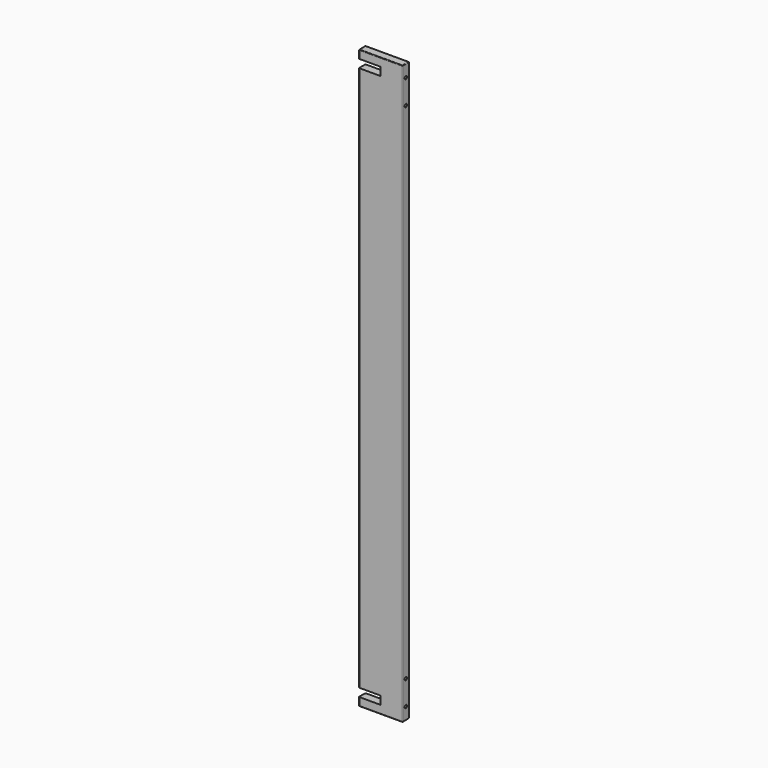
from build123d import *

# Parameters (mm, degrees)
F0_W     = 160
F0_H     = 30
F1_DEPTH = 1060
F2_R     = 2
F3_W     = 2
F3_H     = 30
F3_W_2   = 78
F4_DEPTH = 30.001
F3_W_3   = 80
F3_R     = 5.5
F5_DEPTH = 15
F6_R     = 5.5
F7_DEPTH = 15


# Not quite as in the source:
# - a pattern or mirror of a feature is missing from the dataset's text; its kind, count and spacing are read off the source's solid


with BuildPart() as f1:
    # F0 (on Top) → F1 (new body, symmetric)
    with BuildSketch(Plane.XY):
        Rectangle(F0_W, F0_H)
    extrude(amount=F1_DEPTH, both=True)

    # F2
    f2_edges = [f1.edges().sort_by_distance(p)[0] for p in [
        (0, -15, -1060),
        (80, -15, 0),
        (0, -15, 1060),
        (-80, -15, 0),
        (80, 15, 0),
        (0, 15, -1060),
        (-80, 15, 0),
        (0, 15, 1060),
        (80, 0, 1060),
        (-80, 0, 1060),
        (80, 0, -1060),
        (-80, 0, -1060),
    ]]
    fillet(f2_edges, radius=F2_R)

    # F3 (on face) → F4 (cut, through all)
    with BuildSketch(Plane(origin=(0, 15, 0), x_dir=(-1, 0, 0), z_dir=(0, 1, 0))):
        with Locations((79, 1015)):
            Rectangle(F3_W, F3_H)
        with Locations((39, 1015)):
            Rectangle(F3_W_2, F3_H)
        with Locations((79, -1015)):
            Rectangle(F3_W, F3_H)
        with Locations((39, -1015)):
            Rectangle(F3_W_2, F3_H)
    extrude(amount=-F4_DEPTH, mode=Mode.SUBTRACT)

    # F3 (on face) → F5 (cut)
    with BuildSketch(Plane(origin=(0, 15, 0), x_dir=(-1, 0, 0), z_dir=(0, 1, 0))):
        with Locations((40, 1015)):
            Rectangle(F3_W_3, F3_H)
        with Locations((40, -1015)):
            Rectangle(F3_W_3, F3_H)
        with Locations((25.4589803517, 924.7787594795)):
            Circle(F3_R)
    extrude(amount=-F5_DEPTH, mode=Mode.SUBTRACT)

    # F6 (on face) → F7 (cut)
    with BuildSketch(Plane.YZ.offset(80)):
        with Locations((0, 1015)):
            Circle(F6_R)
        with Locations((0, 925)):
            Circle(F6_R)
    f7 = extrude(amount=-F7_DEPTH, mode=Mode.SUBTRACT)

    # F7_copies: F7 across plane
    add(f7.mirror(Plane(origin=(0, 0, 0), x_dir=(-1, 0, 0), z_dir=(0, 0, -1))), mode=Mode.SUBTRACT)


solid = f1.part
